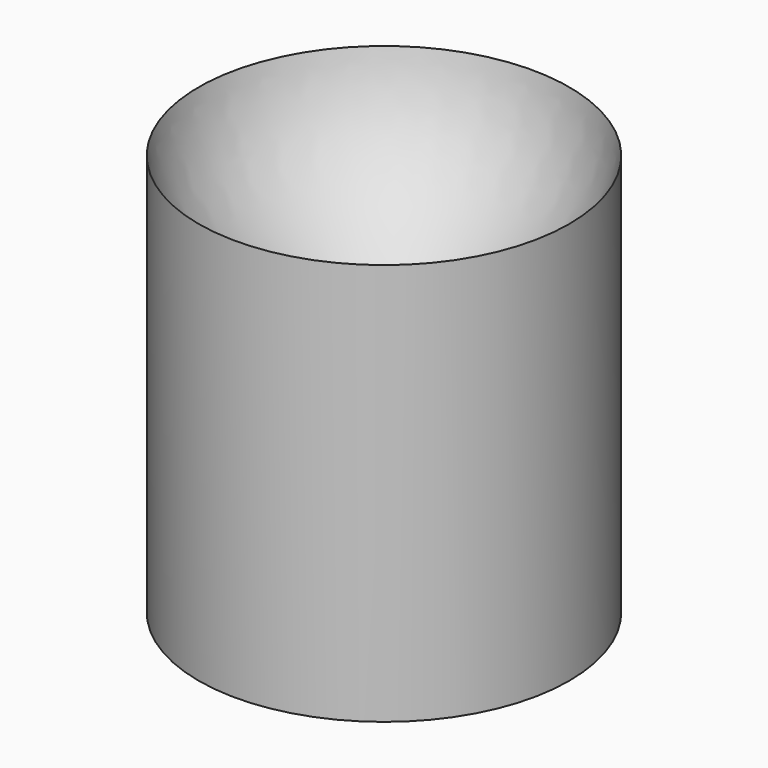
from build123d import *


with BuildPart() as f1:
    # F0 (on Front) → F1 (revolve)
    with BuildSketch(Plane.XZ):
        with BuildLine():
            Line((-20.4611438745, 13.7437874026), (-20.4611438745, 57.5678450522))
            add(Edge.make_bspline(
                [(-20.4611438745, 13.7437874026), (-20.8566771725, 15.9589093815), (-23.4146715047, 24.4188370596), (-37.5810615709, 35.6512550504), (-23.4139334963, 46.8864002179), (-20.8566751777, 55.3496313004), (-20.4611438745, 57.5678450522)],
                knots=[0.188209798, 0.188209798, 0.188209798, 0.188209798, 0.2665049847, 0.5000023645, 0.733494172, 0.8118902995, 0.8118902995, 0.8118902995, 0.8118902995], degree=3))
        make_face()
    revolve(axis=Axis((-40.6541438745, 0, 1.5678450522), (0, 0, -1)))


solid = f1.part
